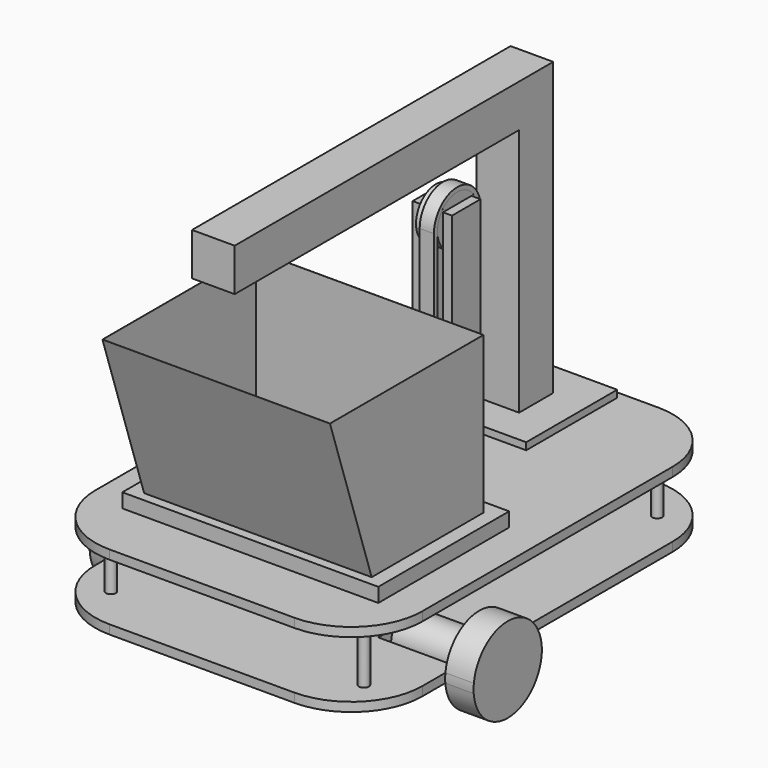
from build123d import *

# Parameters (mm, degrees)
F2_DEPTH  = 6.35
F3_START  = -46.35
F3_DEPTH  = 6.35
F4_R      = 50
F4_2_R    = 50
F6_DEPTH  = 20
F7_R      = 15
F8_DEPTH  = 50
F9_R      = 3.5
F10_DEPTH = 40
F11_W     = 160
F11_H     = 95
F12_DEPTH = 120
F11_W_2   = 80
F11_H_2   = 80
F11_W_3   = 30
F11_H_3   = 30
F13_DEPTH = 5
F15_DEPTH = 160
F16_T     = -0.05
F17_W     = 55
F17_H     = 40
F18_DEPTH = 6.35
F24_DEPTH = 30
F11_W_4   = 180
F11_H_4   = 115
F26_DEPTH = 10
F11_W_5   = 6.35
F11_H_5   = 25
F27_DEPTH = 150
F29_DEPTH = 15
F28_W     = 3
F28_H     = 15.8603712916
F30_DEPTH = 10
F28_W_2   = 2.8027647734
F31_DEPTH = 20


# Not quite as in the source:
# - a feature names something its author has since deleted; it is built from what else it names


with BuildPart() as f2:
    # F0 (on Top) → F2 (new body, through all)
    with BuildSketch(Plane.XY):
        Polygon((0, 70), (0, 0), (230, 0), (230, 70), (230, 130), (230, 320), (0, 320), (0, 130), align=None)
    extrude(amount=-F2_DEPTH)

    # F4
    f4_edges = [f2.edges().sort_by_distance(p)[0] for p in [
        (230, 0, -3.175),
        (230, 320, -3.175),
        (0, 320, -3.175),
        (0, 0, -3.175),
    ]]
    fillet(f4_edges, radius=F4_R)


with BuildPart() as f3:
    # F0 (on Top) → F3 (new body)
    with BuildSketch(Plane.XY.offset(F3_START)):
        Polygon((0, 70), (0, 0), (230, 0), (230, 70), (230, 130), (230, 320), (0, 320), (0, 130), align=None)
    extrude(amount=-F3_DEPTH)

    # F4#2
    f4_2_edges = [f3.edges().sort_by_distance(p)[0] for p in [
        (230, 0, -49.525),
        (230, 320, -49.525),
        (0, 320, -49.525),
        (0, 0, -49.525),
    ]]
    fillet(f4_2_edges, radius=F4_2_R)

    # F17 (on face) → F18 (cut, through all)
    with BuildSketch(Plane(origin=(0, 0, -52.7), x_dir=(1, 0, 0), z_dir=(0, 0, -1))):
        Polygon((0, -80), (0, -85), (0, -115), (0, -120), (55, -120), (55, -80), align=None)
        with Locations((202.5, -100)):
            Rectangle(F17_W, F17_H)
    extrude(amount=-F18_DEPTH, mode=Mode.SUBTRACT)


with BuildPart() as f6:
    # F1 (on Right) → F6 (new body, through all)
    with BuildSketch(Plane.YZ):
        with BuildLine():
            ThreePointArc((70.2228695137, -46.35), (70.0038032651, -49.5223165915), (70.121747039, -52.7))
            Line((70.121747039, -52.7), (129.878252961, -52.7))
            ThreePointArc((129.878252961, -52.7), (129.9695477846, -51.3513717421), (130, -50))
            ThreePointArc((130, -50), (129.9442307848, -48.1716010542), (129.7771304863, -46.35))
            Line((129.7771304863, -46.35), (70.2228695137, -46.35))
        make_face()
        with BuildLine():
            Line((129.878252961, -52.7), (70.121747039, -52.7))
            ThreePointArc((70.121747039, -52.7), (100, -80), (129.878252961, -52.7))
        make_face()
        with BuildLine():
            ThreePointArc((129.7771304863, -46.35), (100, -20), (70.2228695137, -46.35))
            Line((70.2228695137, -46.35), (129.7771304863, -46.35))
        make_face()
    extrude(amount=-F6_DEPTH)


with BuildPart() as f8:
    # F7 (on face) → F8 (new body)
    with BuildSketch(Plane.YZ):
        with Locations((100, -50)):
            Circle(F7_R)
    extrude(amount=F8_DEPTH)


with BuildPart() as f10:
    # F9 (on face) → F10 (new body, through all)
    with BuildSketch(Plane.XY.offset(-46.35)):
        with Locations((26.0077804742, 288.8969213205)):
            Circle(F9_R)
    extrude(amount=F10_DEPTH)


with BuildPart() as f10b:
    # F9 (on face) → F10, piece 2 (new body, through all)
    with BuildSketch(Plane.XY.offset(-46.35)):
        with Locations((26.0077804742, 31.1030786795)):
            Circle(F9_R)
    extrude(amount=F10_DEPTH)


with BuildPart() as f12:
    # F11 (on face) → F12 (new body)
    with BuildSketch(Plane.XY):
        with Locations((115, 100)):
            Rectangle(F11_W, F11_H)
    extrude(amount=F12_DEPTH)

    # F14 (on face) → F15 (join, through all)
    with BuildSketch(Plane.YZ.offset(195)):
        Polygon((12.5, 120), (52.5, 0), (52.5, 120), align=None)
    extrude(amount=-F15_DEPTH)

    # F16
    f16_openings = [f12.faces().sort_by_distance(p)[0] for p in [
        (115, 80, 120),
    ]]
    offset(amount=F16_T, openings=f16_openings)


with BuildPart() as f13:
    # F11 (on face) → F13 (new body)
    with BuildSketch(Plane.XY):
        with Locations((115, 275)):
            Rectangle(F11_W_2, F11_H_2)
        with Locations((115, 275)):
            Rectangle(F11_W_3, F11_H_3, mode=Mode.SUBTRACT)
    extrude(amount=F13_DEPTH)


with BuildPart() as f21:
    # F20 (on plane+point) → F21 (revolve)
    with BuildSketch(Plane.XZ.offset(-290)):
        with BuildLine():
            Line((115, -80), (115, -76))
            Line((115, -76), (108.3667504193, -76))
            ThreePointArc((108.3667504193, -76), (111.1270166538, -78.9226162893), (115, -80))
        make_face()
    revolve(axis=Axis((115, 290, -64.35), (0, 0, -1)))


with BuildPart() as f21b:
    # F20 (on plane+point) → F21, piece 2 (revolve)
    with BuildSketch(Plane.XZ.offset(-290)):
        with BuildLine():
            Line((115, -65), (115, -52.7))
            Line((115, -52.7), (95, -52.7))
            Line((95, -52.7), (95, -55.7))
            Line((95, -55.7), (105, -55.7))
            Line((105, -55.7), (105, -76))
            Line((105, -76), (108.3667504193, -76))
            ThreePointArc((108.3667504193, -76), (108.5773837107, -68.6270166538), (115, -65))
        make_face()
    revolve(axis=Axis((115, 290, -64.35), (0, 0, -1)))


with BuildPart() as f24:
    # F23 (on plane+point) → F24 (new body, through all)
    with BuildSketch(Plane.YZ.offset(130)):
        Polygon((260, 0), (290, 0), (290, 210), (260, 210), (10, 210), (10, 180), (260, 180), align=None)
    extrude(amount=-F24_DEPTH)


with BuildPart() as f25_1:
    # F25: instance of F6
    add(f6.part.mirror(Plane(origin=(115, 160, -3.175), x_dir=(0, -1, 0), z_dir=(-1, 0, 0))))


with BuildPart() as f25_2:
    # F25: instance of F8
    add(f8.part.mirror(Plane(origin=(115, 160, -3.175), x_dir=(0, -1, 0), z_dir=(-1, 0, 0))))


with BuildPart() as f25_3:
    # F25: instance of F10
    add(f10.part.mirror(Plane(origin=(115, 160, -3.175), x_dir=(0, -1, 0), z_dir=(-1, 0, 0))))


with BuildPart() as f25_4:
    # F25: instance of F10b
    add(f10b.part.mirror(Plane(origin=(115, 160, -3.175), x_dir=(0, -1, 0), z_dir=(-1, 0, 0))))


with BuildPart() as f26:
    # F11 (on face) → F26 (new body)
    with BuildSketch(Plane.XY):
        with Locations((115, 100)):
            Rectangle(F11_W_4, F11_H_4)
        with Locations((115, 100)):
            Rectangle(F11_W, F11_H, mode=Mode.SUBTRACT)
        with Locations((115, 100)):
            Rectangle(F11_W, F11_H)
    extrude(amount=F26_DEPTH)


with BuildPart() as f27:
    # F11 (on face) → F27 (new body)
    with BuildSketch(Plane.XY):
        with Locations((125.675, 215)):
            Rectangle(F11_W_5, F11_H_5)
    extrude(amount=F27_DEPTH)


with BuildPart() as f27b:
    # F11 (on face) → F27, piece 2 (new body)
    with BuildSketch(Plane.XY):
        with Locations((104.325, 215)):
            Rectangle(F11_W_5, F11_H_5)
    extrude(amount=F27_DEPTH)


with BuildPart() as f29:
    # F28 (on face) → F29 (new body, through all)
    with BuildSketch(Plane(origin=(122.5, 0, 0), x_dir=(0, -1, 0), z_dir=(-1, 0, 0))):
        with BuildLine():
            ThreePointArc((-202.5, 127.7525512861), (-198.798148254, 133.3856217223), (-197.5, 140))
            ThreePointArc((-197.5, 140), (-215, 157.5), (-232.5, 140))
            ThreePointArc((-232.5, 140), (-231.201851746, 133.3856217223), (-227.5, 127.7525512861))
            Line((-227.5, 127.7525512861), (-227.5, 150))
            Line((-227.5, 150), (-202.5, 150))
            Line((-202.5, 150), (-202.5, 127.7525512861))
        make_face()
        with BuildLine():
            ThreePointArc((-227.5, 127.7525512861), (-215, 122.5), (-202.5, 127.7525512861))
            Line((-202.5, 127.7525512861), (-202.5, 150))
            Line((-202.5, 150), (-227.5, 150))
            Line((-227.5, 150), (-227.5, 127.7525512861))
        make_face()
    extrude(amount=F29_DEPTH)


with BuildPart() as f29b:
    # F28 (on face) → F29, piece 2 (new body, through all)
    with BuildSketch(Plane(origin=(122.5, 0, 0), x_dir=(0, -1, 0), z_dir=(-1, 0, 0))):
        with BuildLine():
            ThreePointArc((-227.5, 52.2474487139), (-231.201851746, 46.6143782777), (-232.5, 40))
            ThreePointArc((-232.5, 40), (-231.201851746, 33.3856217223), (-227.5, 27.7525512861))
            Line((-227.5, 27.7525512861), (-227.5, 52.2474487139))
        make_face()
        with BuildLine():
            Line((-202.5, 27.7525512861), (-202.5, 52.2474487139))
            ThreePointArc((-202.5, 52.2474487139), (-215, 57.5), (-227.5, 52.2474487139))
            Line((-227.5, 52.2474487139), (-227.5, 27.7525512861))
            ThreePointArc((-227.5, 27.7525512861), (-215, 22.5), (-202.5, 27.7525512861))
        make_face()
        with BuildLine():
            ThreePointArc((-197.5, 40), (-198.798148254, 46.6143782777), (-202.5, 52.2474487139))
            Line((-202.5, 52.2474487139), (-202.5, 27.7525512861))
            ThreePointArc((-202.5, 27.7525512861), (-198.798148254, 33.3856217223), (-197.5, 40))
        make_face()
    extrude(amount=F29_DEPTH)


with BuildPart() as f30:
    # F28 (on face) → F30 (new body)
    with BuildSketch(Plane(origin=(122.5, 0, 0), x_dir=(0, -1, 0), z_dir=(-1, 0, 0))):
        with BuildLine():
            ThreePointArc((-232.5, 140), (-215, 157.5), (-197.5, 140))
            Line((-197.5, 140), (-197.5, 82.1528807282))
            Line((-197.5, 82.1528807282), (-194.5, 82.1528807282))
            Line((-194.5, 82.1528807282), (-194.5, 139.999998906))
            ThreePointArc((-194.5, 139.999998906), (-215.0000002942, 160.5), (-235.5, 139.9999983177))
            Line((-235.5, 139.9999983177), (-235.5, 40))
            ThreePointArc((-235.5, 40), (-233.3915741577, 30.9446148619), (-227.5, 23.7519231907))
            Line((-227.5, 23.7519231907), (-227.5, 27.7525512861))
            ThreePointArc((-227.5, 27.7525512861), (-231.201851746, 33.3856217223), (-232.5, 40))
            Line((-232.5, 40), (-232.5, 140))
        make_face()
        with Locations((-196, 74.2226950824)):
            Rectangle(F28_W, F28_H)
        with BuildLine():
            Line((-194.5, 66.2925094366), (-197.5, 66.2925094366))
            Line((-197.5, 66.2925094366), (-197.5, 40))
            ThreePointArc((-197.5, 40), (-198.798148254, 33.3856217223), (-202.5, 27.7525512861))
            Line((-202.5, 27.7525512861), (-202.5, 23.7519231907))
            ThreePointArc((-202.5, 23.7519231907), (-196.6084257123, 30.9446151258), (-194.5, 40.0000005884))
            Line((-194.5, 40.0000005884), (-194.5, 66.2925094366))
        make_face()
        with BuildLine():
            ThreePointArc((-202.5, 27.7525512861), (-215, 22.5), (-227.5, 27.7525512861))
            Line((-227.5, 27.7525512861), (-227.5, 23.7519231907))
            ThreePointArc((-227.5, 23.7519231907), (-215, 19.5), (-202.5, 23.7519231907))
            Line((-202.5, 23.7519231907), (-202.5, 27.7525512861))
        make_face()
    extrude(amount=F30_DEPTH)


with BuildPart() as f31:
    # F28 (on face) → F31 (new body)
    with BuildSketch(Plane(origin=(122.5, 0, 0), x_dir=(0, -1, 0), z_dir=(-1, 0, 0))):
        with Locations((-193.0986176133, 74.2226950824)):
            Rectangle(F28_W_2, F28_H)
        with Locations((-198.9013823867, 74.2226950824)):
            Rectangle(F28_W_2, F28_H)
        with Locations((-196, 74.2226950824)):
            Rectangle(F28_W, F28_H)
        Polygon((-184.7443729639, 82.1528807282), (-191.6972352266, 82.1528807282), (-191.6972352266, 66.2925094366), (-191.6972352266, 0), (-184.7443729639, 0), align=None)
    extrude(amount=F31_DEPTH)


solid = Compound([f2.part, f3.part, f6.part, f8.part, f10.part, f10b.part, f12.part, f13.part, f21.part, f21b.part, f24.part, f25_1.part, f25_2.part, f25_3.part, f25_4.part, f26.part, f27.part, f27b.part, f29.part, f29b.part, f30.part, f31.part])
